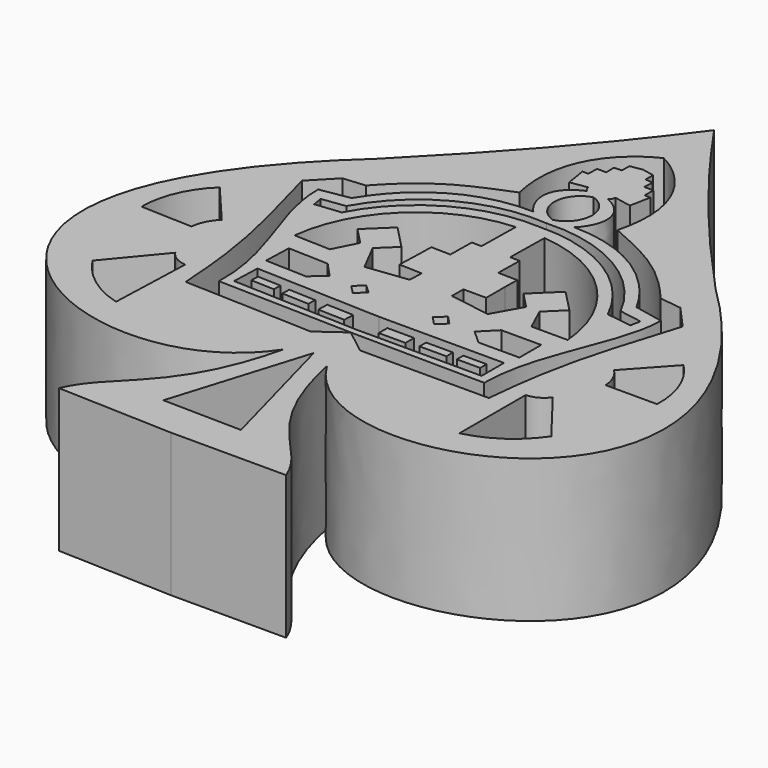
from build123d import *

# Parameters (mm, degrees)
F1_DEPTH = 25.4
F0_W     = 4.128358094
F0_H     = 1.4289282262
F0_W_2   = 4.7634891234
F0_H_2   = 1.468620263
F0_W_3   = 4.7442697883
F0_H_3   = 1.9113573674


# Not quite as in the source:
# - a feature names something its author has since deleted; it is built from what else it names


with BuildPart() as f1:
    # F0 (on Top) → F1 (new body)
    with BuildSketch(Plane.XY):
        with BuildLine():
            Line((-22.9954444695, -37.8900244832), (-2.5283634938, -37.8900244832))
            add(Edge.make_bspline(
                [(-2.5283634938, -37.8900244832), (-5.8608135484, -29.4962804765), (-14.5712196827, -28.3677466214), (-18.5634065419, -8.8018402457)],
                knots=[0, 0, 0, 0, 33.2151331141, 33.2151331141, 33.2151331141, 33.2151331141], degree=3))
            add(Edge.make_bspline(
                [(-18.5634065419, -8.8018402457), (-2.5283634938, -35.3494078415), (62.5428706408, -9.0993279591), (8.9163342491, 43.0122725666)],
                knots=[0, 0, 0, 0, 58.6501358947, 58.6501358947, 58.6501358947, 58.6501358947], degree=3))
            add(Edge.make_bspline(
                [(8.9163342491, 43.0122725666), (-3.4306221642, 56.4400143921), (-11.2726483494, 66.0635232925), (-20.8969525993, 79.9641385674)],
                knots=[0, 0, 0, 0, 47.47917937, 47.47917937, 47.47917937, 47.47917937], degree=3))
            add(Edge.make_bspline(
                [(-52.0068416032, 44.0970606294), (-39.1896790872, 57.0767342864), (-31.0100233031, 66.4149637492), (-20.8969525993, 79.9641385674)],
                knots=[0, 0, 0, 0, 47.47917937, 47.47917937, 47.47917937, 47.47917937], degree=3))
            add(Edge.make_bspline(
                [(-26.3891224094, -8.6624968343), (-43.3591045439, -34.6223823726), (-107.454577438, -6.07238132), (-52.0068416032, 44.0970606294)],
                knots=[0, 0, 0, 0, 58.6501358947, 58.6501358947, 58.6501358947, 58.6501358947], degree=3))
            add(Edge.make_bspline(
                [(-43.4495514732, -37.1613885312), (-39.8203933268, -28.8916017766), (-31.0753324327, -28.0738771005), (-26.3891224094, -8.6624968343)],
                knots=[0, 0, 0, 0, 33.2151331141, 33.2151331141, 33.2151331141, 33.2151331141], degree=3))
            Line((-43.4495514732, -37.1613885312), (-22.9954444695, -37.8900244832))
        make_face()
        Polygon((-29.84915008, -30.9614511052), (-22.4433610347, -6.8842664576), (-15.8994235098, -31.2098376453), (-22.8742867949, -31.0856443752), align=None, mode=Mode.SUBTRACT)
        with BuildLine():
            add(Edge.make_bspline(
                [(-22.3207809169, 0), (-10.655029352, -32.6894562044), (59.6865899861, -11.1531224102), (7.7575119212, 41.9883653522)],
                knots=[0, 0, 0, 0, 51.6500389642, 51.6500389642, 51.6500389642, 51.6500389642], degree=3))
            add(Edge.make_bspline(
                [(-22.3207809169, 0), (-35.1428948343, -32.2534292936), (-104.6732232363, -8.2265585713), (-50.8852053371, 43.0325479438)],
                knots=[0, 0, 0, 0, 51.6500389642, 51.6500389642, 51.6500389642, 51.6500389642], degree=3))
            Line((-50.8852053371, 43.0325479438), (-20.973111277, 75.6869634445))
            Line((-20.973111277, 75.6869634445), (7.7575119212, 41.9883653522))
        make_face(mode=Mode.SUBTRACT)
        with BuildLine():
            add(Edge.make_bspline(
                [(-22.3207809169, 0), (-35.1428948343, -32.2534292936), (-104.6732232363, -8.2265585713), (-50.8852053371, 43.0325479438)],
                knots=[0, 0, 0, 0, 51.6500389642, 51.6500389642, 51.6500389642, 51.6500389642], degree=3))
            add(Edge.make_bspline(
                [(-22.3207809169, 0), (-10.655029352, -32.6894562044), (59.6865899861, -11.1531224102), (7.7575119212, 41.9883653522)],
                knots=[0, 0, 0, 0, 51.6500389642, 51.6500389642, 51.6500389642, 51.6500389642], degree=3))
            Line((7.7575119212, 41.9883653522), (-20.973111277, 75.6869634445))
            Line((-20.973111277, 75.6869634445), (-50.8852053371, 43.0325479438))
        make_face()
        with BuildLine():
            ThreePointArc((-53.4419212435, -11.9822170834), (-59.2752805035, -9.1359017891), (-63.691800004, -4.379438133))
            Line((-63.691800004, -4.379438133), (-56.2167386264, 4.6310161836))
            ThreePointArc((-56.2167386264, 4.6310161836), (-54.7973483092, 3.2789986514), (-52.9181442541, 2.7211345107))
            Line((-52.9181442541, 2.7211345107), (-53.4419212435, -11.9822170834))
        make_face(mode=Mode.SUBTRACT)
        with BuildLine():
            Line((-59.3962358793, 12.1757701265), (-68.5043031466, 12.5002264942))
            ThreePointArc((-68.5043031466, 12.5002264942), (-67.2450849294, 18.6426159936), (-63.6487509213, 23.7788559591))
            Line((-63.6487509213, 23.7788559591), (-57.3389988191, 16.3438184143))
            ThreePointArc((-57.3389988191, 16.3438184143), (-58.7463070002, 14.4467053449), (-59.3962358793, 12.1757701265))
        make_face(mode=Mode.SUBTRACT)
        with BuildLine():
            ThreePointArc((18.8681036234, -5.8494862169), (14.2850517957, -10.4457049841), (8.3540603518, -13.082546182))
            Line((8.3540603518, -13.082546182), (8.3540603518, 1.6301316991))
            ThreePointArc((8.3540603518, 1.6301316991), (10.2519333675, 2.1207418259), (11.7185562849, 3.4213714805))
            Line((11.7185562849, 3.4213714805), (18.8681036234, -5.8494862169))
        make_face(mode=Mode.SUBTRACT)
        with BuildLine():
            ThreePointArc((19.8275279254, 22.2924910486), (23.2387301192, 17.0314760444), (24.2784786969, 10.8481515199))
            Line((24.2784786969, 10.8481515199), (15.1646342129, 10.8481515199))
            ThreePointArc((15.1646342129, 10.8481515199), (14.5959634871, 13.1407849228), (13.2570853457, 15.0867961347))
            Line((13.2570853457, 15.0867961347), (19.8275279254, 22.2924910486))
        make_face(mode=Mode.SUBTRACT)
        with BuildLine():
            add(Edge.make_bspline(
                [(-21.124196495, 69.0203205478), (-22.2645987992, 68.6191021406), (-33.580908588, 63.0681711425), (-30.2861785142, 48.5103170354)],
                knots=[1.924853553, 1.924853553, 1.924853553, 1.924853553, 22.4584134886, 22.4584134886, 22.4584134886, 22.4584134886], degree=3))
            add(Edge.make_bspline(
                [(-21.124196495, 69.0203205478), (-21.1691445632, 69.0500857695), (-21.1554459369, 69.0540761805), (-21.0916213723, 69.0312749979)],
                knots=[0.2728391378, 0.2728391378, 0.2728391378, 0.2728391378, 1.7089042388, 1.7089042388, 1.7089042388, 1.7089042388], degree=3))
            add(Edge.make_bspline(
                [(-21.0594568815, 69.0191678049), (-21.0134776523, 69.04731399), (-21.027025535, 69.0517895479), (-21.0916213723, 69.0312749979)],
                knots=[0.2728391378, 0.2728391378, 0.2728391378, 0.2728391378, 1.7089042388, 1.7089042388, 1.7089042388, 1.7089042388], degree=3))
            add(Edge.make_bspline(
                [(-21.0594568815, 69.0191678049), (-19.9340610017, 68.5776049674), (-8.8225398383, 62.627327695), (-12.633446604, 48.1959953904)],
                knots=[1.924853553, 1.924853553, 1.924853553, 1.924853553, 22.4584134886, 22.4584134886, 22.4584134886, 22.4584134886], degree=3))
            add(Edge.make_bspline(
                [(-12.633446604, 48.1959953904), (-4.4782049954, 44.5908084512), (-1.012446126, 42.8227111697), (4.8599806614, 35.9290093184)],
                knots=[0, 0, 0, 0, 21.3658359252, 21.3658359252, 21.3658359252, 21.3658359252], degree=3))
            Line((4.8599806614, 35.9290093184), (8.7451650402, 35.4348045049))
            Line((8.7451650402, 35.4348045049), (12.5032669737, 31.2499941052))
            add(Edge.make_bspline(
                [(12.5032669737, 31.2499941052), (8.0707731529, 17.1092335792), (6.1978180893, 11.1496476457), (4.9289693125, -2.2719807457)],
                knots=[0, 0, 0, 0, 34.3670304648, 34.3670304648, 34.3670304648, 34.3670304648], degree=3))
            Line((4.9289693125, -2.2719807457), (-17.9089047015, -2.2719807457))
            Line((-17.9089047015, -2.2719807457), (-22.3005021556, 1.1388828675))
            Line((-22.3005021556, 1.1388828675), (-26.8107438558, -2.1134760598))
            Line((-26.8107438558, -2.1134760598), (-49.6341410648, -1.3004389641))
            add(Edge.make_bspline(
                [(-56.0102422262, 32.469934397), (-52.083974651, 18.1803391384), (-50.4243703941, 12.1578530338), (-49.6341410648, -1.3004389641)],
                knots=[0, 0, 0, 0, 34.3670304648, 34.3670304648, 34.3670304648, 34.3670304648], degree=3))
            Line((-56.0102422262, 32.469934397), (-52.105541674, 36.5183021942))
            Line((-52.105541674, 36.5183021942), (-48.2052262113, 36.8738796762))
            add(Edge.make_bspline(
                [(-30.2861785142, 48.5103170354), (-38.5645966004, 45.1977451416), (-42.0911034871, 43.5541509957), (-48.2052262113, 36.8738796762)],
                knots=[0, 0, 0, 0, 21.3658359252, 21.3658359252, 21.3658359252, 21.3658359252], degree=3))
        make_face(mode=Mode.SUBTRACT)
    extrude(amount=F1_DEPTH)


with BuildPart() as f1b:
    # F0 (on Top) → F1, piece 2 (new body)
    with BuildSketch(Plane.XY):
        with BuildLine():
            Line((-46.171825282, 1.7410204233), (-22.3005021556, 1.1388828675))
            Line((-22.3005021556, 1.1388828675), (1.5771253966, 0.8908104501))
            add(Edge.make_bspline(
                [(1.5771253966, 0.8908104501), (1.5829101903, 12.3173911124), (8.8816406205, 21.4957669377), (9.0935900807, 30.7148192078)],
                knots=[0, 0, 0, 0, 30.7566048147, 30.7566048147, 30.7566048147, 30.7566048147], degree=3))
            Line((9.0935900807, 30.7148192078), (3.9008178283, 31.7744798958))
            add(Edge.make_bspline(
                [(3.9008178283, 31.7744798958), (3.0530157965, 33.2580022514), (-3.0935301911, 44.9142754078), (-17.8240444511, 45.1262071729)],
                knots=[0, 0, 0, 0, 25.4997698487, 25.4997698487, 25.4997698487, 25.4997698487], degree=3))
            add(Edge.make_bspline(
                [(-17.8240444511, 45.1262071729), (-15.5544048175, 47.323897481), (-13.9162018895, 51.9864745438), (-19.4513425231, 54.6437501907)],
                knots=[0, 0, 0, 0, 9.6556576219, 9.6556576219, 9.6556576219, 9.6556576219], degree=3))
            add(Edge.make_bspline(
                [(-19.4513425231, 54.6437501907), (-19.084546715, 54.8940747976), (-18.998881802, 55.1322698593), (-18.9135298133, 55.6105002761)],
                knots=[0, 0, 0, 0, 1.1062767458, 1.1062767458, 1.1062767458, 1.1062767458], degree=3))
            Line((-18.9135298133, 55.6105002761), (-15.876889146, 55.0183499966))
            Line((-15.876889146, 55.0183499966), (-15.1645764709, 58.6712025106))
            Line((-15.1645764709, 58.6712025106), (-16.1927435547, 58.6895098848))
            Line((-16.1927435547, 58.6895098848), (-16.1927435547, 60.6039427221))
            Line((-16.1927435547, 60.6039427221), (-17.8136411971, 60.6328041593))
            Line((-17.8136411971, 60.6328041593), (-17.7100636065, 62.3647794127))
            Line((-17.7100636065, 62.3647794127), (-19.0645121038, 62.4766151085))
            Line((-19.0645121038, 62.4766151085), (-19.0645121038, 64.1392618418))
            Line((-19.0645121038, 64.1392618418), (-21.1709695666, 64.5749722779))
            Line((-21.1709695666, 64.5749722779), (-23.2916032165, 64.2145287318))
            Line((-23.2916032165, 64.2145287318), (-23.3507940795, 62.5529359414))
            Line((-23.3507940795, 62.5529359414), (-24.708365393, 62.4893900249))
            Line((-24.708365393, 62.4893900249), (-24.6665124446, 60.7548252592))
            Line((-24.6665124446, 60.7548252592), (-26.287410087, 60.7836866964))
            Line((-26.287410087, 60.7836866964), (-26.355564632, 58.8704674077))
            Line((-26.355564632, 58.8704674077), (-27.3837317159, 58.8887747819))
            Line((-27.3837317159, 58.8887747819), (-26.8019135259, 55.2128791863))
            Line((-26.8019135259, 55.2128791863), (-23.7461169911, 55.6965485296))
            add(Edge.make_bspline(
                [(-23.2430618726, 54.7112649227), (-23.6007135185, 54.974488922), (-23.6778442933, 55.2155826969), (-23.7461169911, 55.6965485296)],
                knots=[0, 0, 0, 0, 1.1062767458, 1.1062767458, 1.1062767458, 1.1062767458], degree=3))
            add(Edge.make_bspline(
                [(-25.2081565999, 45.257687461), (-27.3981189013, 47.5347847087), (-28.8692938451, 52.2527268432), (-23.2430618726, 54.7112649227)],
                knots=[0, 0, 0, 0, 9.6556576219, 9.6556576219, 9.6556576219, 9.6556576219], degree=3))
            add(Edge.make_bspline(
                [(-47.394574231, 32.6878372218), (-46.4944956501, 34.1402371022), (-39.9368781188, 45.5703020096), (-25.2081565999, 45.257687461)],
                knots=[0, 0, 0, 0, 25.4997698487, 25.4997698487, 25.4997698487, 25.4997698487], degree=3))
            Line((-47.394574231, 32.6878372218), (-52.6217791411, 31.8137129357))
            add(Edge.make_bspline(
                [(-46.171825282, 1.7410204233), (-45.7708157439, 13.1605637788), (-52.73816584, 22.5929590908), (-52.6217791411, 31.8137129357)],
                knots=[0, 0, 0, 0, 30.7566048147, 30.7566048147, 30.7566048147, 30.7566048147], degree=3))
        make_face()
        Polygon((-44.7576590216, 15.5055557954), (-37.679395917, 15.2534070716), (-35.1471528411, 12.5197675079), (-37.679395917, 10.3981904904), (-44.9303970315, 10.6564926543), align=None, mode=Mode.SUBTRACT)
        Polygon((-30.9412721545, 12.0524866506), (-29.4437312744, 13.5210845619), (-27.8865820009, 12.0524866506), (-29.4437312744, 10.525432397), align=None, mode=Mode.SUBTRACT)
        Polygon((-44.3688373522, 8.0533013785), (-22.1914521969, 7.263277148), (0, 7.263277148), (0, 2.287469827), (-22.2800506048, 2.287469827), (-44.5459780059, 3.0806481949), align=None, mode=Mode.SUBTRACT)
        Polygon((-14.8276363188, 10.2651806109), (-16.3294348053, 11.8467019859), (-14.72098995, 13.2589338481), (-13.2766810033, 11.7379538419), align=None, mode=Mode.SUBTRACT)
        Polygon((-9.0568310236, 12.0552075228), (-6.4288745034, 14.6969654201), (0.65387832, 14.6969654201), (0.65387832, 9.8448265344), (-6.6017220804, 9.8448265344), align=None, mode=Mode.SUBTRACT)
        with BuildLine():
            Line((-40.1418328888, 18.7965188536), (-46.5573088461, 19.0250571336))
            ThreePointArc((-46.5573088461, 19.0250571336), (-39.2386461395, 33.6660544705), (-24.1943614945, 40.115172732))
            Line((-24.1943614945, 40.115172732), (-24.3272148478, 32.6539473716))
            Line((-24.3272148478, 32.6539473716), (-26.0486511449, 32.6845989835))
            Line((-26.0486511449, 32.6845989835), (-26.1316949705, 28.0207445723))
            Line((-26.1316949705, 28.0207445723), (-29.55665306, 28.0817288135))
            Line((-29.55665306, 28.0817288135), (-29.6034895982, 25.4513250038))
            Line((-29.6034895982, 25.4513250038), (-29.7527835425, 21.2603784792))
            Line((-29.7527835425, 21.2603784792), (-25.7005311791, 21.1160252323))
            Line((-25.7005311791, 21.1160252323), (-25.7912743076, 18.568704235))
            Line((-25.7912743076, 18.568704235), (-33.0961882413, 17.6953475839))
            Line((-33.0961882413, 17.6953475839), (-35.7368813782, 22.7922350813))
            Line((-35.7368813782, 22.7922350813), (-32.84917873, 25.5710387789))
            Line((-32.84917873, 25.5710387789), (-36.9155790608, 29.7967978759))
            Line((-36.9155790608, 29.7967978759), (-40.934720905, 25.9292229978))
            Line((-40.934720905, 25.9292229978), (-38.0526815829, 22.9342390088))
            Line((-38.0526815829, 22.9342390088), (-40.1418328888, 18.7965188536))
        make_face(mode=Mode.SUBTRACT)
        with BuildLine():
            ThreePointArc((-21.5435338647, 43.6512536062), (-7.2201754113, 40.2072674631), (2.8851975221, 29.4880755246))
            Line((2.8851975221, 29.4880755246), (6.9841672666, 28.7952069193))
            Line((6.9841672666, 28.7952069193), (6.6132862121, 26.9937831908))
            Line((6.6132862121, 26.9937831908), (2.1097264253, 27.6295803487))
            ThreePointArc((2.1097264253, 27.6295803487), (-7.5677131963, 38.4280486782), (-21.5694110126, 42.1979577158))
            ThreePointArc((-21.5694110126, 42.1979577158), (-35.6964434395, 38.9289042288), (-45.7521782087, 28.4818015615))
            Line((-45.7521782087, 28.4818015615), (-50.2755178366, 28.006735892))
            Line((-50.2755178366, 28.006735892), (-50.5820324143, 29.8202212158))
            Line((-50.5820324143, 29.8202212158), (-46.4609945958, 30.3667257165))
            ThreePointArc((-46.4609945958, 30.3667257165), (-35.9804200494, 40.7193676554), (-21.5435338647, 43.6512536062))
        make_face(mode=Mode.SUBTRACT)
        with BuildLine():
            Line((-19.1531257722, 32.5618183913), (-19.0202724189, 40.0230437517))
            ThreePointArc((-19.0202724189, 40.0230437517), (-4.2151153543, 33.0424312338), (2.5776829571, 18.1501675397))
            Line((2.5776829571, 18.1501675397), (-3.8418623153, 18.1501675397))
            Line((-3.8418623153, 18.1501675397), (-5.7823848911, 22.3596394062))
            Line((-5.7823848911, 22.3596394062), (-2.7955498966, 25.250123183))
            Line((-2.7955498966, 25.250123183), (-6.6744568758, 29.2583294213))
            Line((-6.6744568758, 29.2583294213), (-10.888718186, 25.1800144253))
            Line((-10.888718186, 25.1800144253), (-8.101772517, 22.3001688719))
            Line((-8.101772517, 22.3001688719), (-10.9222428873, 17.3005219549))
            Line((-10.9222428873, 17.3005219549), (-18.191434443, 18.4333827347))
            Line((-18.191434443, 18.4333827347), (-18.191434443, 20.9823194891))
            Line((-18.191434443, 20.9823194891), (-14.1366117494, 20.9823194891))
            Line((-14.1366117494, 20.9823194891), (-14.1366117494, 25.1759243172))
            Line((-14.1366117494, 25.1759243172), (-14.0897752112, 27.8063281269))
            Line((-14.0897752112, 27.8063281269), (-17.5147333007, 27.8673123681))
            Line((-17.5147333007, 27.8673123681), (-17.4316894751, 32.5311667793))
            Line((-17.4316894751, 32.5311667793), (-19.1531257722, 32.5618183913))
        make_face(mode=Mode.SUBTRACT)
        with BuildLine():
            ThreePointArc((-21.3630149606, 53.7894412541), (-18.12483498, 49.3327404002), (-21.5196225597, 44.9941450771))
            ThreePointArc((-21.5196225597, 44.9941450771), (-24.7578025403, 49.4508459311), (-21.3630149606, 53.7894412541))
        make_face(mode=Mode.SUBTRACT)
    extrude(amount=F1_DEPTH)


with BuildPart() as f1c:
    # F0 (on Top) → F1, piece 3 (new body)
    with BuildSketch(Plane.XY):
        with Locations((-3.7132945145, 4.7373422422)):
            Rectangle(F0_W, F0_H)
    extrude(amount=F1_DEPTH)


with BuildPart() as f1d:
    # F0 (on Top) → F1, piece 4 (new body)
    with BuildSketch(Plane.XY):
        with Locations((-9.8661344964, 4.5587262139)):
            Rectangle(F0_W_2, F0_H_2)
    extrude(amount=F1_DEPTH)


with BuildPart() as f1e:
    # F0 (on Top) → F1, piece 5 (new body)
    with BuildSketch(Plane.XY):
        with Locations((-16.7828049063, 4.3770501642)):
            Rectangle(F0_W_3, F0_H_3)
    extrude(amount=F1_DEPTH)


with BuildPart() as f1f:
    # F0 (on Top) → F1, piece 6 (new body)
    with BuildSketch(Plane.XY):
        Polygon((-25.3628130835, 3.5319078526), (-25.2947680263, 5.4420536208), (-30.0360304476, 5.6109514494), (-30.1040755048, 3.7008056811), align=None)
    extrude(amount=F1_DEPTH)


with BuildPart() as f1g:
    # F0 (on Top) → F1, piece 7 (new body)
    with BuildSketch(Plane.XY):
        Polygon((-32.2511469345, 4.1805909847), (-32.1988634885, 5.6482802973), (-36.9593330619, 5.8178623416), (-37.011616508, 4.350173029), align=None)
    extrude(amount=F1_DEPTH)


with BuildPart() as f1h:
    # F0 (on Top) → F1, piece 8 (new body)
    with BuildSketch(Plane.XY):
        Polygon((-38.7103855509, 4.6092761508), (-38.6595151567, 6.0372985872), (-42.7852563068, 6.1842697226), (-42.8361267011, 4.7562472863), align=None)
    extrude(amount=F1_DEPTH)


solid = Compound([f1.part, f1b.part, f1c.part, f1d.part, f1e.part, f1f.part, f1g.part, f1h.part])
